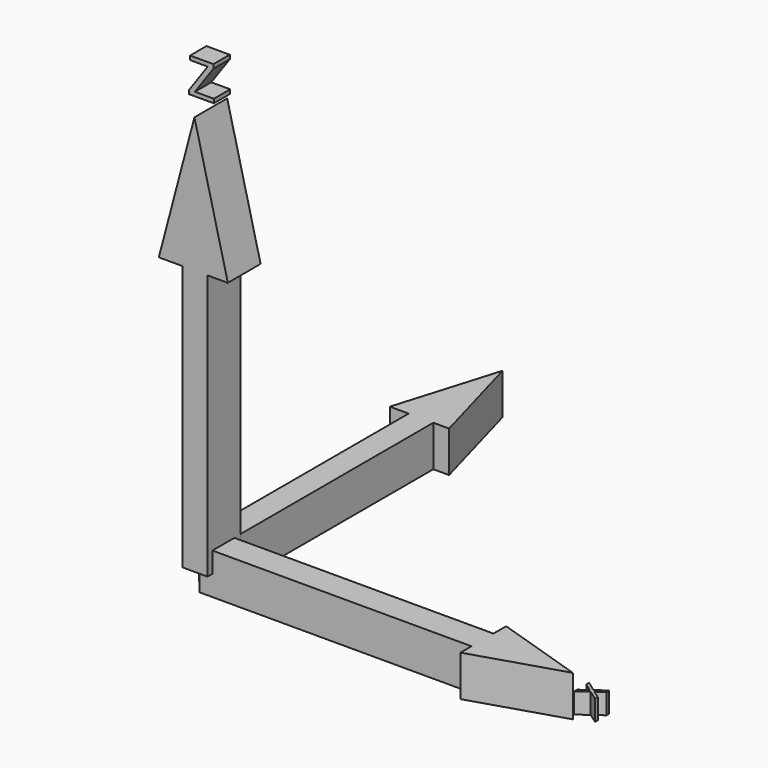
from build123d import *

# Parameters (mm, degrees)
F2_DEPTH     = 2
F4_DEPTH     = 2
F5_TEXT_SIZE = 6.2675991406
F6_DEPTH     = 1
F9_TEXT_SIZE = 3.7285201769
F10_DEPTH    = 1


# Not quite as in the source:
# - ends of sketch curves that miss each other by under 0.0002 mm in the source are joined
# - the program builds the solid bodies; features that only make, move or delete a surface that nothing else refers to are left out
# - Text() gives the source's letters only with a copy of the font that has no kerning and outlines rounded to 1/6400 em; it was checked with that copy


with BuildPart() as f2:
    # F0 (on Top) → F2 (new body, symmetric)
    with BuildSketch(Plane.XY):
        Polygon((-1.1715167202, 25.6020948291), (-1.1715167202, 0), (1.2434370583, 0), (1.2434370583, 25.6020950474), (2.7823126903, 25.6020950474), (0, 35.5996489525), (-3.0052513571, 25.6020950474), align=None)
    extrude(amount=F2_DEPTH, both=True)


with BuildPart() as f2b:
    # F1 (on Top) → F2, piece 2 (new body, symmetric)
    with BuildSketch(Plane.XY):
        Polygon((0, 1.2810530607), (0, 0), (0, -1.4021554962), (26.5696421266, -1.4021554962), (26.5696421266, -2.7438503396), (35.3510528803, 0), (26.5696421266, 2.8356104735), (26.5696421266, 1.2810530607), align=None)
    extrude(amount=F2_DEPTH, both=True)


with BuildPart() as f4:
    # F3 (on Front) → F4 (new body, symmetric)
    with BuildSketch(Plane.XZ):
        Polygon((-1.1607919587, 0), (0, 0), (1.2784901774, 0), (1.2784901774, 25.8988365531), (3.2612838211, 25.8988365531), (0, 39.0709526837), (-3.4781098366, 25.8988365531), (-1.1607919587, 25.8988365531), align=None)
    extrude(amount=F4_DEPTH, both=True)


with BuildPart() as f6:
    # F5 (on Front) → F6 (new body, symmetric)
    with BuildSketch(Plane.XZ):
        with Locations((-1.588342071, 40.2173064649)):
            Text('z', F5_TEXT_SIZE, font='Open Sans', text_align=(TextAlign.LEFT, TextAlign.BOTTOM))
    extrude(amount=F6_DEPTH, both=True)


with BuildPart() as f10:
    # F9 (on Top) → F10 (new body, symmetric)
    with BuildSketch(Plane.XY):
        with Locations(Location((36.1319312158, 1.0677970511), (0, 0, -90))):
            Text('x', F9_TEXT_SIZE, font='Open Sans', text_align=(TextAlign.LEFT, TextAlign.BOTTOM))
    extrude(amount=F10_DEPTH, both=True)


solid = Compound([f2.part, f2b.part, f4.part, f6.part, f10.part])
